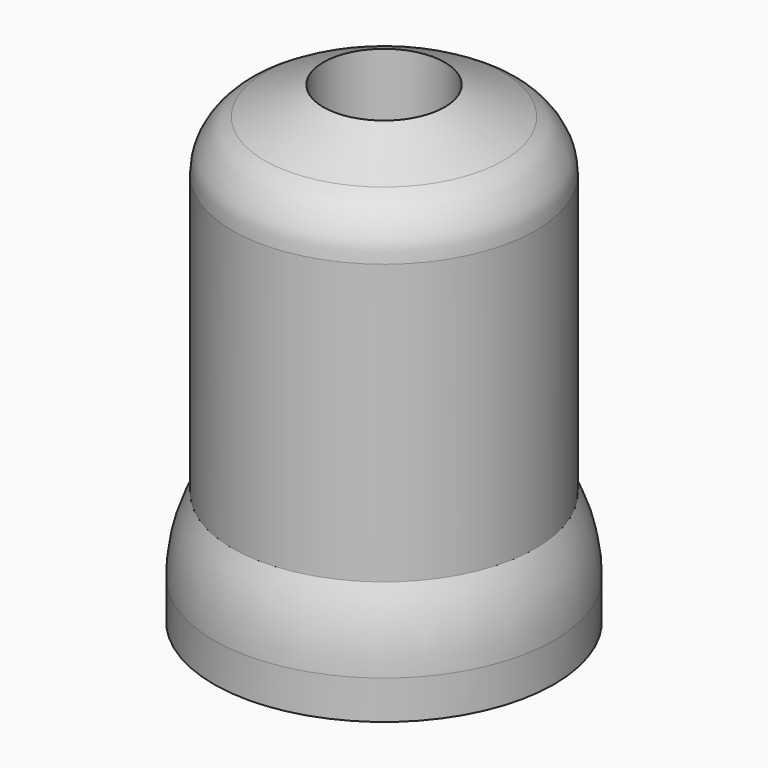
from build123d import *

# Parameters (mm, degrees)
F2_R     = 2.7
F3_DEPTH = 44.201
F4_R     = 11.6
F4_R_2   = 7.75
F5_DEPTH = 38.2
F6_R     = 5
F8_R     = 5.35
F9_DEPTH = 34.1


# Not quite as in the source:
# - a fillet or chamfer that OpenCascade refuses, or shapes differently, is made with other operations: its cross-section is extruded or revolved along the edge and cut away or added


with BuildPart() as f1:
    # F0 (on Front) → F1 (revolve)
    with BuildSketch(Plane.XZ):
        Polygon((0, -25.2708706191), (0, 18.9291293809), (-13.35, 12.5291293809), (-13.35, -15.2708706191), (-15, -15.2708706191), (-15, -25.2708706191), align=None)
    revolve(axis=Axis((0, 0, -3.1708706191), (0, 0, -1)))

    # F2 (on face) → F3 (cut, through all)
    with BuildSketch(Plane(origin=(0, 0, -25.2708706191), x_dir=(1, 0, 0), z_dir=(0, 0, -1))):
        Circle(F2_R)
    extrude(amount=-F3_DEPTH, mode=Mode.SUBTRACT)

    # F4 (on face) → F5 (cut)
    with BuildSketch(Plane(origin=(0, 0, -25.2708706191), x_dir=(1, 0, 0), z_dir=(0, 0, -1))):
        Circle(F4_R)
        Circle(F4_R_2, mode=Mode.SUBTRACT)
    extrude(amount=-F5_DEPTH, mode=Mode.SUBTRACT)

    # F6
    f6_edges = [f1.edges().sort_by_distance(p)[0] for p in [
        (13.35, 0, 12.529129),
    ]]
    fillet(f6_edges, radius=F6_R)

    # F8 (on offset) → F9 (cut)
    with BuildSketch(Plane.XY.offset(17.8)):
        Circle(F8_R)
    extrude(amount=-F9_DEPTH, mode=Mode.SUBTRACT)

    # F10: fillet of radius 14 on 1 edges, made by hand

    # F10_s1 → F10_t2 (revolve, cut)
    with BuildSketch(Plane.XZ):
        with BuildLine():
            ThreePointArc((-13.35, -15.2708706191), (-14.5812370571, -18.4660885634), (-15, -21.864617657))
            Line((-15, -21.864617657), (-15, -15.2708706191))
            Line((-15, -15.2708706191), (-13.35, -15.2708706191))
        make_face()
    revolve(axis=Axis((0, 0, -15.2708706191), (0, 0, -1)), mode=Mode.SUBTRACT)


solid = f1.part
